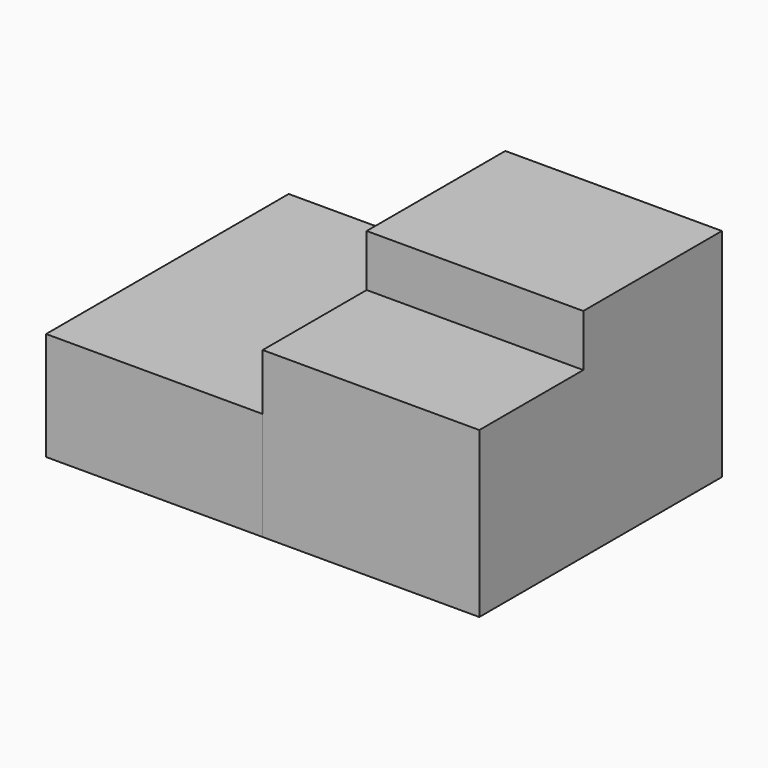
from build123d import *

# Parameters (mm, degrees)
F1_W     = 1270
F1_H     = 965.2
F2_DEPTH = 1778
F0_W     = 1270
F0_H     = 635
F3_DEPTH = 1778
F6_W     = 1270
F6_H     = 1016
F7_DEPTH = 304.8


# Not quite as in the source:
# - a feature of the source that left no trace in its solid (it failed there, or was rolled back) is left out


with BuildPart() as f2:
    # F1 (on Front) → F2 (new body)
    with BuildSketch(Plane.XZ):
        with Locations((142.6505839825, -584.8500465393)):
            Rectangle(F1_W, F1_H)
    extrude(amount=F2_DEPTH)

    # F6 (on face) → F7 (join)
    with BuildSketch(Plane.XY.offset(-102.2500465393)):
        with Locations((142.6505839825, -508)):
            Rectangle(F6_W, F6_H)
    extrude(amount=F7_DEPTH)


with BuildPart() as f3:
    # F0 (on Front) → F3 (new body)
    with BuildSketch(Plane.XZ):
        with Locations((-1127.3534202576, -749.9475431442)):
            Rectangle(F0_W, F0_H)
    extrude(amount=F3_DEPTH)


solid = Compound([f2.part, f3.part])
